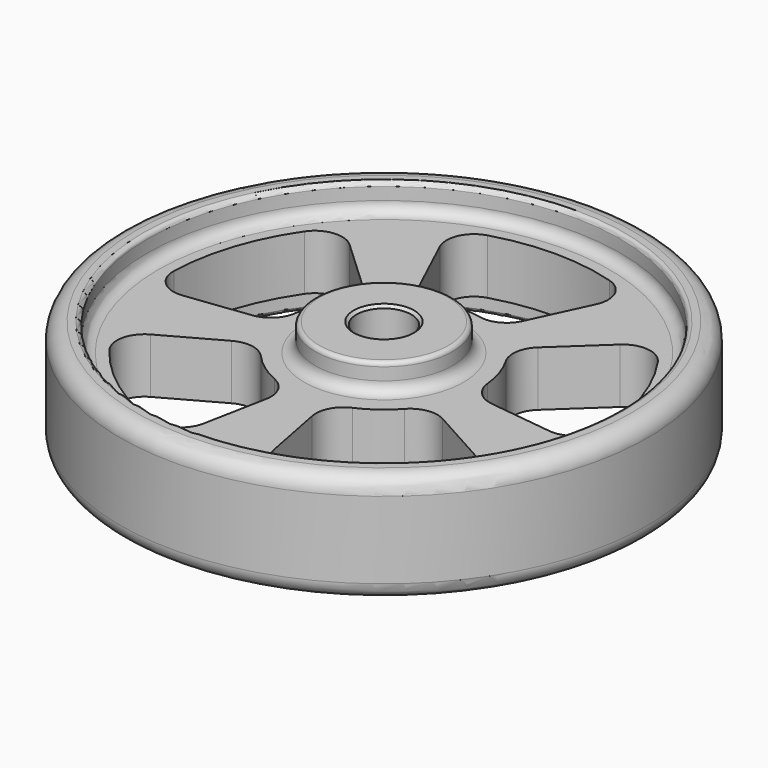
from build123d import *

# Parameters (mm, degrees)
F2_R            = 2
F3_R            = 3
F4_SIZE         = 0.5
F5_R            = 0.75
F8_DEPTH        = 20.001
F8_COPIES_COUNT = 5


# Not quite as in the source:
# - a pattern or mirror of a feature is missing from the dataset's text; its kind, count and spacing are read off the source's solid
# - a feature names something its author has since deleted; it is built from what else it names


with BuildPart() as f1:
    # F0 (on Front) → F1 (revolve)
    with BuildSketch(Plane.XZ):
        Polygon((-5, -20), (-5, 0), (-12.5, 0), (-12.5, -5), (-43, -5), (-43, 0), (-48, 0), (-48, -20), (-43, -20), (-43, -15), (-12.5, -15), (-12.5, -20), align=None)
    revolve(axis=Axis((0, 0, -8.972), (0, 0, -1)))

    # F2
    f2_edges = [f1.edges().sort_by_distance(p)[0] for p in [
        (12.5, 0, -5),
        (43, 0, -5),
        (12.5, 0, -15),
        (43, 0, -15),
    ]]
    fillet(f2_edges, radius=F2_R)

    # F3
    f3_edges = [f1.edges().sort_by_distance(p)[0] for p in [
        (48, 0, 0),
        (48, 0, -20),
    ]]
    fillet(f3_edges, radius=F3_R)

    # F4
    f4_edges = [f1.edges().sort_by_distance(p)[0] for p in [
        (12.5, 0, -20),
        (5, 0, -20),
        (5, 0, 0),
        (-5, 0, -10),
    ]]
    chamfer(f4_edges, length=F4_SIZE)

    # F5
    f5_edges = [f1.edges().sort_by_distance(p)[0] for p in [
        (-43, 0, -18.5),
        (43, 0, -17),
        (43, 0, -20),
        (-43, 0, -1.5),
        (43, 0, -3),
        (43, 0, 0),
        (12.5, 0, 0),
    ]]
    fillet(f5_edges, radius=F5_R)

    # F6 (on Top) → F8 (cut, through all)
    with BuildSketch(Plane.XY):
        with BuildLine():
            ThreePointArc((-11.1049728154, 37.3855530756), (-14.2408474581, 34.6443977691), (-14.212797287, 30.4794421418))
            Line((-14.212797287, 30.4794421418), (-9.2711504906, 19.8820463882))
            ThreePointArc((-9.2711504906, 19.8820463882), (-6.9643345444, 17.5173472124), (-3.6863645431, 17.1073293198))
            ThreePointArc((-3.6863645431, 17.1073293198), (0, 17.5), (3.6863645431, 17.1073293198))
            ThreePointArc((3.6863645431, 17.1073293198), (6.9643345444, 17.5173472124), (9.2711504906, 19.8820463882))
            Line((9.2711504906, 19.8820463882), (14.212797287, 30.4794421418))
            ThreePointArc((14.212797287, 30.4794421418), (14.2408474581, 34.6443977691), (11.1049728154, 37.3855530756))
            ThreePointArc((11.1049728154, 37.3855530756), (0, 39), (-11.1049728154, 37.3855530756))
        make_face()
    f8 = extrude(amount=-F8_DEPTH, mode=Mode.SUBTRACT)

    # F8_copies: F8 ×5 about axis
    f8_copies_axis = Axis((0, 0, 0), (0, 0, 1))
    for i in range(1, F8_COPIES_COUNT):
        add(f8.rotate(f8_copies_axis, i * 360 / F8_COPIES_COUNT), mode=Mode.SUBTRACT)


solid = f1.part
